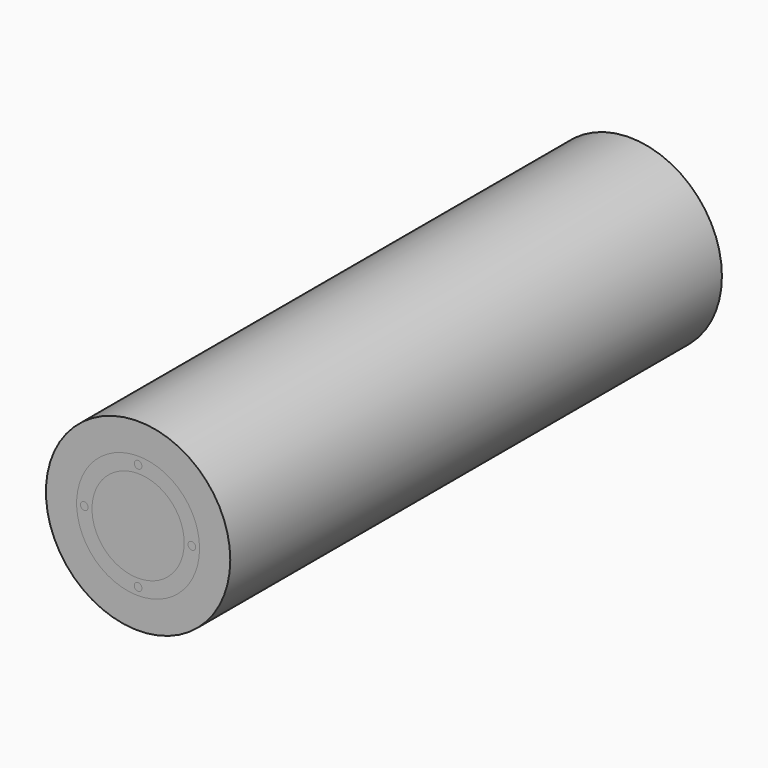
from build123d import *

# Parameters (mm, degrees)
F2_R      = 38.1
F2_R_2    = 25.4
F4_DEPTH  = 254
F1_R      = 25.4
F1_R_2    = 19.05
F5_DEPTH  = 254
F6_START  = -25.4
F0_R      = 19.05
F6_DEPTH  = 228.6
F3_R      = 1.5875
F7_DEPTH  = 254
F8_DEPTH  = 254
F12_DEPTH = 254


with BuildPart() as f4:
    # F2 (on Front) → F4 (new body)
    with BuildSketch(Plane.XZ):
        Circle(F2_R)
        Circle(F2_R_2, mode=Mode.SUBTRACT)
    extrude(amount=-F4_DEPTH)


with BuildPart() as f5:
    # F1 (on Front) → F5 (new body)
    with BuildSketch(Plane.XZ):
        Circle(F1_R)
        Circle(F1_R_2, mode=Mode.SUBTRACT)
    extrude(amount=-F5_DEPTH)


with BuildPart() as f6:
    # F0 (on Front) → F6 (new body)
    with BuildSketch(Plane.XZ.offset(F6_START)):
        Circle(F0_R)
    extrude(amount=-F6_DEPTH)

    # F0 (on Front) → F8 (join)
    with BuildSketch(Plane.XZ):
        Circle(F0_R)
    extrude(amount=-F8_DEPTH)


with BuildPart() as f7:
    # F3 (on Front) → F7 (new body)
    with BuildSketch(Plane.XZ):
        with Locations((0, 22.225)):
            Circle(F3_R)
    extrude(amount=-F7_DEPTH)


with BuildPart() as f7b:
    # F3 (on Front) → F7, piece 2 (new body)
    with BuildSketch(Plane.XZ):
        with Locations((-22.225, 0)):
            Circle(F3_R)
    extrude(amount=-F7_DEPTH)


with BuildPart() as f7c:
    # F3 (on Front) → F7, piece 3 (new body)
    with BuildSketch(Plane.XZ):
        with Locations((22.225, -0.042203279)):
            Circle(F3_R)
    extrude(amount=-F7_DEPTH)


with BuildPart() as f7d:
    # F3 (on Front) → F7, piece 4 (new body)
    with BuildSketch(Plane.XZ):
        with Locations((0, -22.225)):
            Circle(F3_R)
    extrude(amount=-F7_DEPTH)


with BuildPart() as f10_1:
    # F10: copy of F7b
    add(f7b.part)


with BuildPart() as f12:
    # F0 (on Front) → F12 (new body)
    with BuildSketch(Plane.XZ):
        Circle(F0_R)
    extrude(amount=-F12_DEPTH)


solid = Compound([f4.part, f5.part, f7.part, f7b.part, f7c.part, f7d.part, f12.part])
